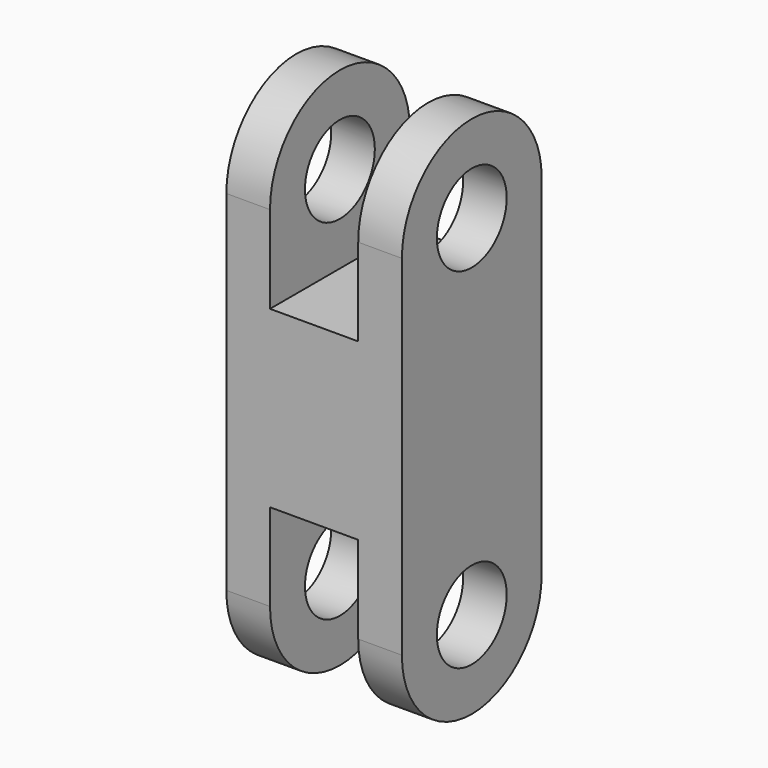
from build123d import *

# Parameters (mm, degrees)
F0_W     = 40
F0_H     = 80
F1_DEPTH = 20.1
F2_R     = 10
F3_DEPTH = 10
F5_W     = 20.2
F5_H     = 40
F6_DEPTH = 40
F7_R     = 10
F8_DEPTH = 40.2
F9_R     = 19.99999


# Not quite as in the source:
# - a fillet or chamfer is up to 0.001 mm smaller than in the source, because OpenCascade refuses the exact size


with BuildPart() as f1:
    # F0 (on Right) → F1 (new body)
    with BuildSketch(Plane.YZ):
        Rectangle(F0_W, F0_H)
    extrude(amount=F1_DEPTH)

    # F2 (on face) → F3 (join)
    with BuildSketch(Plane.YZ.offset(20.1)):
        with BuildLine():
            Line((-20, 60), (-20, 40))
            Line((-20, 40), (20, 40))
            Line((20, 40), (20, 60))
            ThreePointArc((20, 60), (0, 80), (-20, 60))
        make_face()
        with Locations((0, 60)):
            Circle(F2_R, mode=Mode.SUBTRACT)
    extrude(amount=-F3_DEPTH)

    # F4: F1 across plane


with BuildPart() as f1_1:
    add(f1.part)
    add(f1.part.mirror(Plane.YZ))

    # F5 (on face) → F6 (cut, through all)
    with BuildSketch(Plane.XZ.offset(20)):
        with Locations((0, -20)):
            Rectangle(F5_W, F5_H)
    extrude(amount=-F6_DEPTH, mode=Mode.SUBTRACT)

    # F7 (on face) → F8 (cut, through all)
    with BuildSketch(Plane.YZ.offset(20.1)):
        with Locations((0, -20)):
            Circle(F7_R)
    extrude(amount=-F8_DEPTH, mode=Mode.SUBTRACT)

    # F9 (radius 20 in the source; OpenCascade refuses exactly that, so slightly less here)
    f9_edges = [f1_1.edges().sort_by_distance(p)[0] for p in [
        (15.1, 20, -40),
        (-15.1, 20, -40),
        (15.1, -20, -40),
        (-15.1, -20, -40),
    ]]
    fillet(f9_edges, radius=F9_R)


solid = f1_1.part
